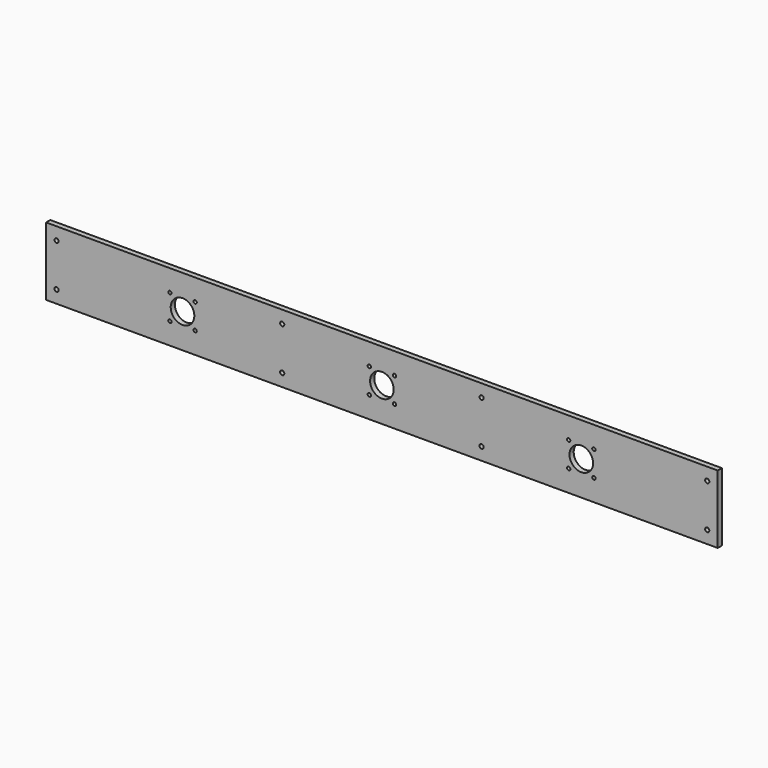
from build123d import *

# Parameters (mm, degrees)
F0_W     = 812.8
F0_H     = 82.55
F1_DEPTH = 6.35
F3_DEPTH = 6.35
F5_DEPTH = 6.35


# Not quite as in the source:
# - a pattern or mirror of a feature is missing from the dataset's text; its kind, count and spacing are read off the source's solid


with BuildPart() as f1:
    # F0 (on Front) → F1 (new body)
    with BuildSketch(Plane.XZ):
        Rectangle(F0_W, F0_H)
    extrude(amount=F1_DEPTH)

    # F2 (on face) → F3 (cut, through all)
    with BuildSketch(Plane.XZ.offset(6.35)):
        with BuildLine():
            ThreePointArc((-254.508, 15.24), (-257.9768409794, 16.6768409794), (-256.54, 13.208))
            Line((-256.54, 13.208), (-256.54, 15.24))
            Line((-256.54, 15.24), (-254.508, 15.24))
        make_face()
        with BuildLine():
            Line((-256.54, 15.24), (-256.54, 13.208))
            ThreePointArc((-256.54, 13.208), (-255.1031590206, 13.8031590206), (-254.508, 15.24))
            Line((-254.508, 15.24), (-256.54, 15.24))
        make_face()
        with BuildLine():
            Line((-241.3, 0), (-255.5875, 0))
            ThreePointArc((-255.5875, 0), (-241.3, -14.2875), (-227.0125, 0))
            ThreePointArc((-227.0125, 0), (-231.1972118638, 10.1027881362), (-241.3, 14.2875))
            Line((-241.3, 14.2875), (-241.3, 0))
        make_face()
        with BuildLine():
            ThreePointArc((-241.3, 14.2875), (-251.4027881362, 10.1027881362), (-255.5875, 0))
            Line((-255.5875, 0), (-241.3, 0))
            Line((-241.3, 0), (-241.3, 14.2875))
        make_face()
        with BuildLine():
            Line((-256.54, -15.24), (-256.54, -13.208))
            ThreePointArc((-256.54, -13.208), (-257.9768409794, -16.6768409794), (-254.508, -15.24))
            Line((-254.508, -15.24), (-256.54, -15.24))
        make_face()
        with BuildLine():
            ThreePointArc((-254.508, -15.24), (-255.1031590206, -13.8031590206), (-256.54, -13.208))
            Line((-256.54, -13.208), (-256.54, -15.24))
            Line((-256.54, -15.24), (-254.508, -15.24))
        make_face()
        with BuildLine():
            Line((-226.06, -15.24), (-228.092, -15.24))
            ThreePointArc((-228.092, -15.24), (-226.06, -17.272), (-224.028, -15.24))
            ThreePointArc((-224.028, -15.24), (-224.6231590206, -13.8031590206), (-226.06, -13.208))
            Line((-226.06, -13.208), (-226.06, -15.24))
        make_face()
        with BuildLine():
            ThreePointArc((-226.06, -13.208), (-227.4968409794, -13.8031590206), (-228.092, -15.24))
            Line((-228.092, -15.24), (-226.06, -15.24))
            Line((-226.06, -15.24), (-226.06, -13.208))
        make_face()
        with BuildLine():
            ThreePointArc((-224.028, 15.24), (-227.4968409794, 16.6768409794), (-226.06, 13.208))
            ThreePointArc((-226.06, 13.208), (-224.6231590206, 13.8031590206), (-224.028, 15.24))
        make_face()
        with BuildLine():
            ThreePointArc((14.2875, 0), (10.1027881362, 10.1027881362), (0, 14.2875))
            ThreePointArc((0, 14.2875), (-10.1027881362, -10.1027881362), (14.2875, 0))
        make_face()
        with BuildLine():
            Line((15.24, -15.24), (13.208, -15.24))
            ThreePointArc((13.208, -15.24), (15.24, -17.272), (17.272, -15.24))
            ThreePointArc((17.272, -15.24), (16.6768409794, -13.8031590206), (15.24, -13.208))
            Line((15.24, -13.208), (15.24, -15.24))
        make_face()
        with BuildLine():
            ThreePointArc((15.24, -13.208), (13.8031590206, -13.8031590206), (13.208, -15.24))
            Line((13.208, -15.24), (15.24, -15.24))
            Line((15.24, -15.24), (15.24, -13.208))
        make_face()
        with BuildLine():
            ThreePointArc((17.272, 15.24), (13.8031590206, 16.6768409794), (15.24, 13.208))
            ThreePointArc((15.24, 13.208), (16.6768409794, 13.8031590206), (17.272, 15.24))
        make_face()
        with BuildLine():
            Line((-15.24, 15.24), (-13.208, 15.24))
            ThreePointArc((-13.208, 15.24), (-16.6768409794, 16.6768409794), (-15.24, 13.208))
            Line((-15.24, 13.208), (-15.24, 15.24))
        make_face()
        with BuildLine():
            ThreePointArc((-15.24, 13.208), (-13.8031590206, 13.8031590206), (-13.208, 15.24))
            Line((-13.208, 15.24), (-15.24, 15.24))
            Line((-15.24, 15.24), (-15.24, 13.208))
        make_face()
        with BuildLine():
            Line((-15.24, -15.24), (-15.24, -13.208))
            ThreePointArc((-15.24, -13.208), (-16.6768409794, -16.6768409794), (-13.208, -15.24))
            Line((-13.208, -15.24), (-15.24, -15.24))
        make_face()
        with BuildLine():
            ThreePointArc((-13.208, -15.24), (-13.8031590206, -13.8031590206), (-15.24, -13.208))
            Line((-15.24, -13.208), (-15.24, -15.24))
            Line((-15.24, -15.24), (-13.208, -15.24))
        make_face()
    f3 = extrude(amount=-F3_DEPTH, mode=Mode.SUBTRACT)

    # F3_copies: F3 across plane
    add(f3.mirror(Plane(origin=(120.65, 0, 0), x_dir=(0, 0, 1), z_dir=(1, 0, 0))), mode=Mode.SUBTRACT)

    # F4 (on face) → F5 (cut, through all)
    with BuildSketch(Plane.XZ.offset(6.35)):
        with BuildLine():
            ThreePointArc((-391.16, 26.035), (-391.9039487758, 27.8310512242), (-393.7, 28.575))
            Line((-393.7, 28.575), (-393.7, 23.495))
            ThreePointArc((-393.7, 23.495), (-391.9039487758, 24.2389487758), (-391.16, 26.035))
        make_face()
        with BuildLine():
            ThreePointArc((-391.16, -26.035), (-391.9039487758, -24.2389487758), (-393.7, -23.495))
            Line((-393.7, -23.495), (-393.7, -28.575))
            ThreePointArc((-393.7, -28.575), (-391.9039487758, -27.8310512242), (-391.16, -26.035))
        make_face()
        with BuildLine():
            Line((-393.7, -28.575), (-393.7, -23.495))
            ThreePointArc((-393.7, -23.495), (-396.24, -26.035), (-393.7, -28.575))
        make_face()
        with BuildLine():
            Line((-393.7, 23.495), (-393.7, 28.575))
            ThreePointArc((-393.7, 28.575), (-396.24, 26.035), (-393.7, 23.495))
        make_face()
        with BuildLine():
            ThreePointArc((-118.11, 26.035), (-118.8539487758, 27.8310512242), (-120.65, 28.575))
            Line((-120.65, 28.575), (-120.65, 23.495))
            ThreePointArc((-120.65, 23.495), (-118.8539487758, 24.2389487758), (-118.11, 26.035))
        make_face()
        with BuildLine():
            ThreePointArc((-118.11, -26.035), (-118.8539487758, -24.2389487758), (-120.65, -23.495))
            Line((-120.65, -23.495), (-120.65, -28.575))
            ThreePointArc((-120.65, -28.575), (-118.8539487758, -27.8310512242), (-118.11, -26.035))
        make_face()
        with BuildLine():
            Line((-120.65, -28.575), (-120.65, -23.495))
            ThreePointArc((-120.65, -23.495), (-123.19, -26.035), (-120.65, -28.575))
        make_face()
        with BuildLine():
            Line((-120.65, 23.495), (-120.65, 28.575))
            ThreePointArc((-120.65, 28.575), (-123.19, 26.035), (-120.65, 23.495))
        make_face()
    f5 = extrude(amount=-F5_DEPTH, mode=Mode.SUBTRACT)

    # F5_copies: F5 across plane
    add(f5.mirror(Plane(origin=(0, 0, 0), x_dir=(0, 0, 1), z_dir=(1, 0, 0))), mode=Mode.SUBTRACT)


solid = f1.part
